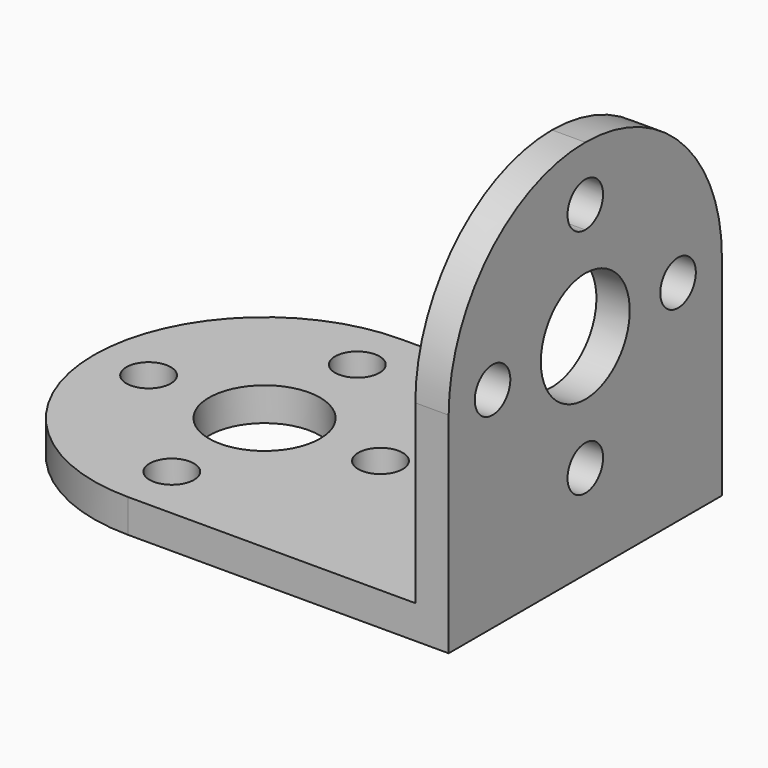
from build123d import *

# Parameters (mm, degrees)
F0_W     = 35.4
F0_H     = 24.6
F1_DEPTH = 2.4
F2_W     = 2.4
F2_H     = 24.6
F3_DEPTH = 25
F4_R     = 12.29999
F5_R     = 1.6
F6_DEPTH = 3
F7_R     = 1.6
F8_DEPTH = 3


# Not quite as in the source:
# - a fillet or chamfer is up to 0.001 mm smaller than in the source, because OpenCascade refuses the exact size


with BuildPart() as f1:
    # F0 (on Top) → F1 (new body)
    with BuildSketch(Plane.XY):
        Rectangle(F0_W, F0_H)
    extrude(amount=F1_DEPTH)

    # F2 (on face) → F3 (join)
    with BuildSketch(Plane.XY.offset(2.4)):
        with Locations((16.5, 0)):
            Rectangle(F2_W, F2_H)
    extrude(amount=F3_DEPTH)

    # F4 (radius 12.3 in the source; OpenCascade refuses exactly that, so slightly less here)
    f4_edges = [f1.edges().sort_by_distance(p)[0] for p in [
        (16.5, -12.3, 27.4),
        (16.5, 12.3, 27.4),
        (-17.7, -12.3, 1.2),
        (-17.7, 12.3, 1.2),
    ]]
    fillet(f4_edges, radius=F4_R)

    # F5 (on face) → F6 (cut)
    with BuildSketch(Plane(origin=(15.3, 0, 0), x_dir=(0, -1, 0), z_dir=(-1, 0, 0))):
        with BuildLine():
            ThreePointArc((0, 19.1), (-2.8284271247, 12.2715728753), (4, 15.1))
            ThreePointArc((4, 15.1), (2.8284271247, 17.9284271247), (0, 19.1))
        make_face()
        with BuildLine():
            ThreePointArc((1.6, 23.45), (-1.1313708499, 24.5813708499), (0, 21.85))
            ThreePointArc((0, 21.85), (1.1313708499, 22.3186291501), (1.6, 23.45))
        make_face()
        with Locations((-8.35, 15.1)):
            Circle(F5_R)
        with Locations((0, 6.75)):
            Circle(F5_R)
        with Locations((8.35, 15.1)):
            Circle(F5_R)
    extrude(amount=-F6_DEPTH, mode=Mode.SUBTRACT)

    # F7 (on face) → F8 (cut)
    with BuildSketch(Plane.XY.offset(2.4)):
        with BuildLine():
            ThreePointArc((-9.4, 0), (-5.4, -4), (-1.4, 0))
            ThreePointArc((-1.4, 0), (-5.4, 4), (-9.4, 0))
        make_face()
        with Locations((-13.75, 0)):
            Circle(F7_R)
        with Locations((-5.4, -8.35)):
            Circle(F7_R)
        with Locations((2.95, 0)):
            Circle(F7_R)
        with Locations((-5.4, 8.35)):
            Circle(F7_R)
    extrude(amount=-F8_DEPTH, mode=Mode.SUBTRACT)


solid = f1.part
